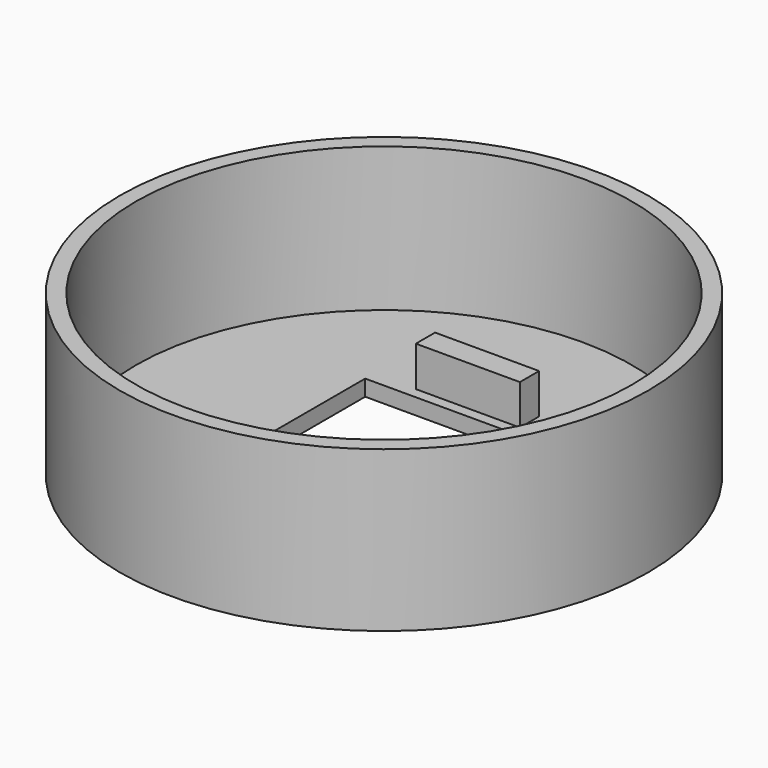
from build123d import *

# Parameters (mm, degrees)
F0_R     = 33
F1_DEPTH = 20
F2_T     = -2
F3_DEPTH = 102
F4_W     = 23.5
F4_H     = 23.5
F5_DEPTH = 12.5
F6_W     = 13
F6_H     = 3
F6_H_2   = 2.9999976491
F7_DEPTH = 7


# Not quite as in the source:
# - an extrude ends at something that could not be found from the text; its depth is read off the source's solid


with BuildPart() as f1:
    # F0 (on Top) → F1 (new body)
    with BuildSketch(Plane.XY):
        Circle(F0_R)
    extrude(amount=F1_DEPTH)

    # F2
    f2_openings = [f1.faces().sort_by_distance(p)[0] for p in [
        (0, 0, 20),
    ]]
    offset(amount=F2_T, openings=f2_openings)

    # F0 (on Top) → F3 (cut, through all)
    with BuildSketch(Plane.XY):
        Circle(F0_R)
    extrude(amount=-F3_DEPTH, mode=Mode.SUBTRACT)

    # F4 (on face) → F5 (cut, symmetric)
    with BuildSketch(Plane.XY):
        Rectangle(F4_W, F4_H)
    extrude(amount=F5_DEPTH, both=True, mode=Mode.SUBTRACT)

    # F6 (on Top) → F7 (join)
    with BuildSketch(Plane.XY):
        with Locations((0, 14.5980315283)):
            Rectangle(F6_W, F6_H)
        with Locations((0, -14.5859429613)):
            Rectangle(F6_W, F6_H_2)
    extrude(amount=F7_DEPTH)


solid = f1.part
